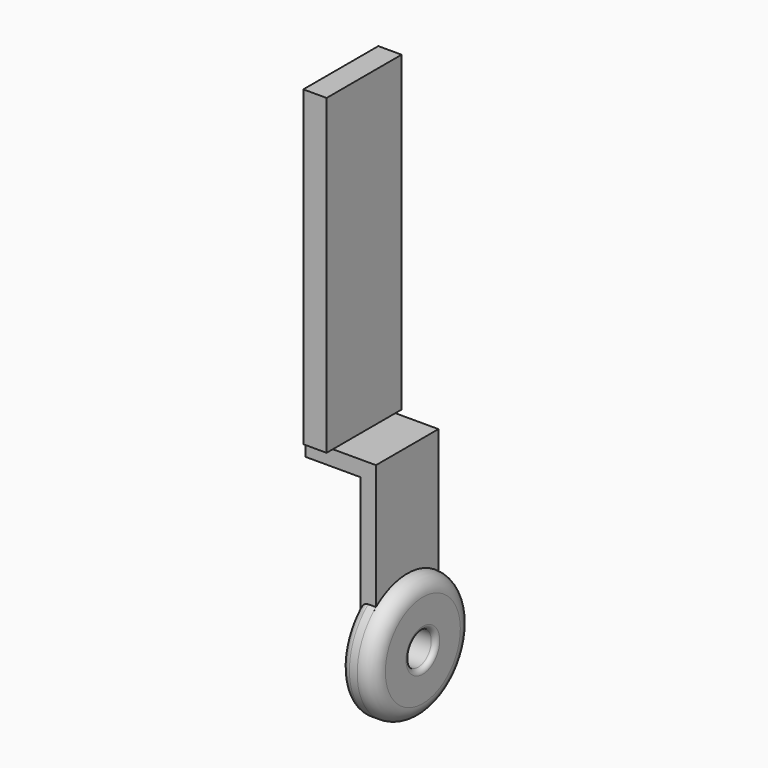
from build123d import *

# Parameters (mm, degrees)
F0_R      = 10.16
F1_DEPTH  = 2.54
F2_R      = 2.667
F3_DEPTH  = 26.02296
F4_R      = 10.16
F5_DEPTH  = 5.08
F7_R      = 2.667
F8_DEPTH  = 61.29661
F9_DEPTH  = 2.54
F10_W     = 8.89
F10_H     = 12.7
F11_DEPTH = 2.54
F13_DEPTH = 50.8
F14_R     = 2.53999
F15_R     = 1.27
F16_R     = 0.762


# Not quite as in the source:
# - a fillet or chamfer is up to 0.001 mm smaller than in the source, because OpenCascade refuses the exact size


with BuildPart() as f1:
    # F0 (on Right) → F1 (new body)
    with BuildSketch(Plane.YZ):
        Circle(F0_R)
    extrude(amount=-F1_DEPTH)

    # F2 (on face) → F3 (cut)
    with BuildSketch(Plane(origin=(-2.54, 0, 0), x_dir=(0, -1, 0), z_dir=(-1, 0, 0))):
        Circle(F2_R)
    extrude(amount=-F3_DEPTH, mode=Mode.SUBTRACT)

    # F4 (on Right) → F5 (join)
    with BuildSketch(Plane.YZ):
        Circle(F4_R)
    extrude(amount=-F5_DEPTH)

    # F7 (on face) → F8 (cut)
    with BuildSketch(Plane(origin=(-5.08, 0, 0), x_dir=(0, -1, 0), z_dir=(-1, 0, 0))):
        Circle(F7_R)
    extrude(amount=-F8_DEPTH, mode=Mode.SUBTRACT)

    # F6 (on face) → F9 (join)
    with BuildSketch(Plane(origin=(-5.08, 0, 0), x_dir=(0, -1, 0), z_dir=(-1, 0, 0))):
        with BuildLine():
            Line((-6.35, 28.251147458), (-6.35, 7.931147458))
            ThreePointArc((-6.35, 7.931147458), (0, 10.16), (6.35, 7.931147458))
            Line((6.35, 7.931147458), (6.35, 28.251147458))
            Line((6.35, 28.251147458), (-6.35, 28.251147458))
        make_face()
    extrude(amount=-F9_DEPTH)

    # F10 (on face) → F11 (join)
    with BuildSketch(Plane.XY.offset(28.251147458)):
        with Locations((-9.525, 0)):
            Rectangle(F10_W, F10_H)
    extrude(amount=-F11_DEPTH)

    # F12 (on face) → F13 (join)
    with BuildSketch(Plane.XY.offset(28.251147458)):
        Polygon((-9.5504, 7.62), (-13.335, 7.62), (-13.335, -7.62), (-9.5504, -7.62), (-9.5504, 0), align=None)
    extrude(amount=F13_DEPTH)

    # F14 (radius 2.54 in the source; OpenCascade refuses exactly that, so slightly less here)
    f14_edges = [f1.edges().sort_by_distance(p)[0] for p in [
        (0, -10.16, 0),
    ]]
    fillet(f14_edges, radius=F14_R)

    # F15
    f15_edges = [f1.edges().sort_by_distance(p)[0] for p in [
        (-5.08, -4.399409, -9.1581),
    ]]
    fillet(f15_edges, radius=F15_R)

    # F16
    f16_edges = [f1.edges().sort_by_distance(p)[0] for p in [
        (-5.08, 2.667, 0),
        (0, 2.667, 0),
    ]]
    fillet(f16_edges, radius=F16_R)


solid = f1.part
